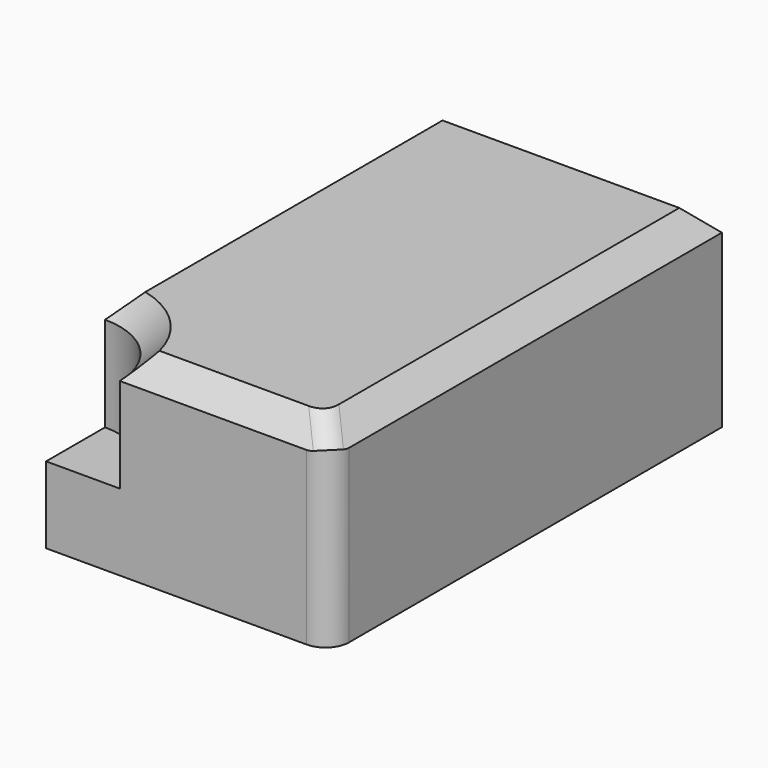
from build123d import *

# Parameters (mm, degrees)
F0_W     = 59.9947497249
F0_H     = 41.1609634757
F1_DEPTH = 103.378
F3_DEPTH = 25
F4_SIZE  = 5
F5_F1_R  = 5
F5_F2_R  = 5


with BuildPart() as f1:
    # F0 (on Front) → F1 (new body)
    with BuildSketch(Plane.XZ):
        with Locations((29.9973748624, 20.5804817379)):
            Rectangle(F0_W, F0_H)
    extrude(amount=F1_DEPTH)

    # F2 (on face) → F3 (cut)
    with BuildSketch(Plane.XY.offset(41.1609634757)):
        with BuildLine():
            ThreePointArc((0, -87.8144259489), (-11.005108751, -114.383108751), (15.5635740511, -103.378))
            Line((15.5635740511, -103.378), (0, -103.378))
            Line((0, -103.378), (0, -87.8144259489))
        make_face()
        with BuildLine():
            Line((0, -103.378), (15.5635740511, -103.378))
            ThreePointArc((15.5635740511, -103.378), (11.005108751, -92.372891249), (0, -87.8144259489))
            Line((0, -87.8144259489), (0, -103.378))
        make_face()
    extrude(amount=-F3_DEPTH, mode=Mode.SUBTRACT)

    # F4
    f4_edges = [f1.edges().sort_by_distance(p)[0] for p in [
        (29.997375, 0, 41.160963),
        (0, -43.907213, 41.160963),
        (11.005109, -92.372891, 41.160963),
        (37.779162, -103.378, 41.160963),
        (59.99475, -51.689, 41.160963),
    ]]
    chamfer(f4_edges, length=F4_SIZE)

    # F5: fillet of radius 5 on 2 edges, made by hand

    # F5_f1
    f5_f1_edges = [f1.edges().sort_by_distance(p)[0] for p in [
        (59.9947497249, -103.378, 18.0804817379),
    ]]
    fillet(f5_f1_edges, radius=F5_F1_R)

    # F5_f2
    f5_f2_edges = [f1.edges().sort_by_distance(p)[0] for p in [
        (56.7625166778, -100.145766953, 39.3931965227),
    ]]
    fillet(f5_f2_edges, radius=F5_F2_R)


solid = f1.part
